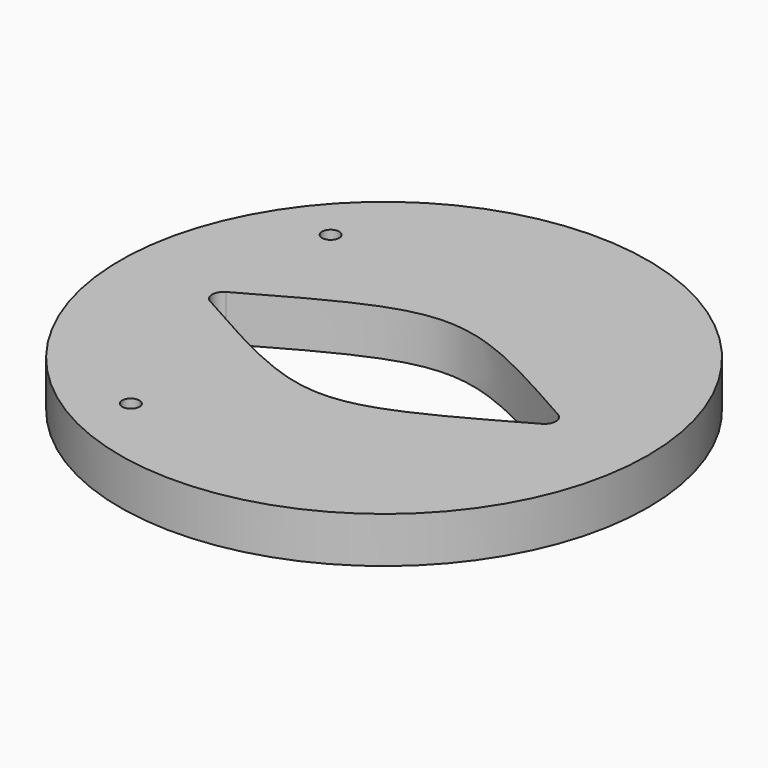
from build123d import *

# Parameters (mm, degrees)
F0_R     = 115
F1_DEPTH = 20
F2_R     = 5
F3_R     = 3.7625
F4_DEPTH = 25


with BuildPart() as f1:
    # F0 (on Top) → F1 (new body)
    with BuildSketch(Plane.XY):
        Circle(F0_R)
        with BuildLine():
            add(Edge.make_bspline(
                [(-80, 0), (0, -45.502603054), (0, -45.502603054), (80, 0)],
                knots=[0, 0, 0, 0, 160, 160, 160, 160], degree=3))
            add(Edge.make_bspline(
                [(-80, 0), (0, 45.502603054), (0, 45.502603054), (80, 0)],
                knots=[0, 0, 0, 0, 160, 160, 160, 160], degree=3))
        make_face(mode=Mode.SUBTRACT)
    extrude(amount=F1_DEPTH)

    # F2
    f2_edges = [f1.edges().sort_by_distance(p)[0] for p in [
        (-80, 0, 10),
        (80, 0, 10),
    ]]
    fillet(f2_edges, radius=F2_R)

    # F3 (on Top) → F4 (cut)
    with BuildSketch(Plane.XY):
        with Locations((-70.8591109885, 59.457853896)):
            Circle(F3_R)
        with Locations((-46.25, -80.1073498501)):
            Circle(F3_R)
    extrude(amount=F4_DEPTH, mode=Mode.SUBTRACT)


solid = f1.part
